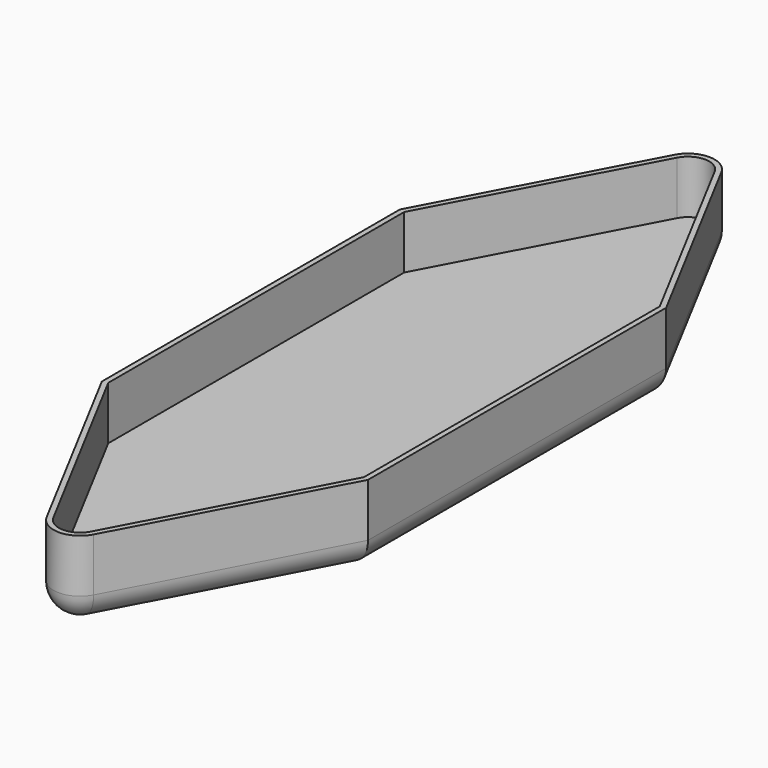
from build123d import *

# Parameters (mm, degrees)
F1_DEPTH     = 381
F2_R         = 127
F3_T1_DEPTH  = 1430.9172960673
F3_T3_DEPTH  = 2413
F3_T5_DEPTH  = 1430.9172960673
F3_T7_DEPTH  = 850.9
F3_T12_DEPTH = 127
F3_T18_DEPTH = 127
F5_DEPTH     = 254


# Not quite as in the source:
# - a fillet or chamfer that OpenCascade refuses, or shapes differently, is made with other operations: its cross-section is extruded or revolved along the edge and cut away or added


with BuildPart() as f1:
    # F0 (on Top) → F1 (new body)
    with BuildSketch(Plane.XY):
        Polygon((-635, 0), (0, 0), (0, 2082.8), (-635, 889), align=None)
        Polygon((635, 0), (0, 0), (-635, 0), (-635, -889), (0, -2082.8), (635, -889), align=None)
        Polygon((0, 2082.8), (0, 0), (635, 0), (635, 889), align=None)
    extrude(amount=F1_DEPTH)

    # F2
    f2_edges = [f1.edges().sort_by_distance(p)[0] for p in [
        (635, 0, 0),
        (317.5, -1485.9, 0),
        (317.5, 1485.9, 0),
    ]]
    fillet(f2_edges, radius=F2_R)

    # F3: fillet of radius 127 on 3 edges, made by hand

    # F3_s2 → F3_t1 (cut)
    with BuildSketch(Plane(origin=(751.4214309895, 1412.6722902602, 0), x_dir=(0, 0, 1), z_dir=(-0.469612973, -0.8828723892, 0))):
        with BuildLine():
            ThreePointArc((127, 978.1099001193), (37.1974387893, 940.91246133), (0, 851.1099001193))
            Line((0, 851.1099001193), (0, 978.1099001193))
            Line((0, 978.1099001193), (127, 978.1099001193))
        make_face()
    extrude(amount=F3_T1_DEPTH, mode=Mode.SUBTRACT)

    # F3_s4 → F3_t3 (cut)
    with BuildSketch(Plane.XZ.offset(-1206.5)):
        with BuildLine():
            ThreePointArc((-508, 0), (-597.8025612107, 37.1974387893), (-635, 127))
            Line((-635, 127), (-635, 0))
            Line((-635, 0), (-508, 0))
        make_face()
    extrude(amount=F3_T3_DEPTH, mode=Mode.SUBTRACT)

    # F3_s6 → F3_t5 (cut)
    with BuildSketch(Plane(origin=(79.4441054972, -149.3549183347, 0), x_dir=(0, 0, 1), z_dir=(0.469612973, -0.8828723892, 0))):
        with BuildLine():
            ThreePointArc((0, 851.1099001193), (37.1974387893, 940.91246133), (127, 978.1099001193))
            Line((127, 978.1099001193), (0, 978.1099001193))
            Line((0, 978.1099001193), (0, 851.1099001193))
        make_face()
    extrude(amount=F3_T5_DEPTH, mode=Mode.SUBTRACT)

    # F3_s8 → F3_t7 (cut)
    with BuildSketch(Plane.XY.offset(127)):
        with BuildLine():
            ThreePointArc((-112.1247934283, -1872.0053883548), (0, -1939.3645407865), (112.1247934283, -1872.0053883548))
            Line((112.1247934283, -1872.0053883548), (0, -2082.8))
            Line((0, -2082.8), (-112.1247934283, -1872.0053883548))
        make_face()
        with BuildLine():
            ThreePointArc((-112.1247934283, 1872.0053883548), (0, 1939.3645407865), (112.1247934283, 1872.0053883548))
            Line((112.1247934283, 1872.0053883548), (0, 2082.8))
            Line((0, 2082.8), (-112.1247934283, 1872.0053883548))
        make_face()
    extrude(amount=F3_T7_DEPTH, mode=Mode.SUBTRACT)


with BuildPart() as f3_tool10:
    # F3_s11 → F3_t12 (new body)
    with BuildSketch(Plane.XY.offset(127)):
        Polygon((0, -1812.3645407865), (-112.1247934283, -1872.0053883548), (0, -2082.8), (112.1247934283, -1872.0053883548), align=None)
    extrude(amount=-F3_T12_DEPTH)

    # F3_s13 → F3_t14 (revolve, cut)
    with BuildSketch(Plane(origin=(0, -1812.3645407865, 127), x_dir=(0, 1, 0), z_dir=(-1, 0, 0))):
        with BuildLine():
            ThreePointArc((0, -127), (127, 0), (0, 127))
            Line((0, 127), (0, -127))
        make_face()
    revolve(axis=Axis((0, -1812.3645407865, 127), (0, 0, -1)), mode=Mode.SUBTRACT)


with BuildPart() as f1_1:
    add(f1.part)

    # F3_t9: cut F3_tool10
    add(f3_tool10.part, mode=Mode.SUBTRACT)


with BuildPart() as f3_tool16:
    # F3_s17 → F3_t18 (new body)
    with BuildSketch(Plane.XY.offset(127)):
        Polygon((0, 1812.3645407865), (-112.1247934283, 1872.0053883548), (0, 2082.8), (112.1247934283, 1872.0053883548), align=None)
    extrude(amount=-F3_T18_DEPTH)

    # F3_s19 → F3_t20 (revolve, cut)
    with BuildSketch(Plane(origin=(0, 1812.3645407865, 127), x_dir=(0, -1, 0), z_dir=(1, 0, 0))):
        with BuildLine():
            ThreePointArc((0, -127), (127, 0), (0, 127))
            Line((0, 127), (0, -127))
        make_face()
    revolve(axis=Axis((0, 1812.3645407865, 127), (0, 0, -1)), mode=Mode.SUBTRACT)


with BuildPart() as f1_2:
    add(f1_1.part)

    # F3_t15: cut F3_tool16
    add(f3_tool16.part, mode=Mode.SUBTRACT)

    # F4 (on face) → F5 (cut)
    with BuildSketch(Plane.XY.offset(381)):
        with BuildLine():
            Line((-609.6, -882.6649081573), (-89.6998347426, -1860.0772188411))
            ThreePointArc((-89.6998347426, -1860.0772188411), (0, -1913.9645407865), (89.6998347426, -1860.0772188411))
            Line((89.6998347426, -1860.0772188411), (609.6, -882.6649081573))
            Line((609.6, -882.6649081573), (609.6, 882.6649081573))
            Line((609.6, 882.6649081573), (89.6998347426, 1860.0772188411))
            ThreePointArc((89.6998347426, 1860.0772188411), (0, 1913.9645407865), (-89.6998347426, 1860.0772188411))
            Line((-89.6998347426, 1860.0772188411), (-609.6, 882.6649081573))
            Line((-609.6, 882.6649081573), (-609.6, -882.6649081573))
        make_face()
    extrude(amount=-F5_DEPTH, mode=Mode.SUBTRACT)


solid = f1_2.part
